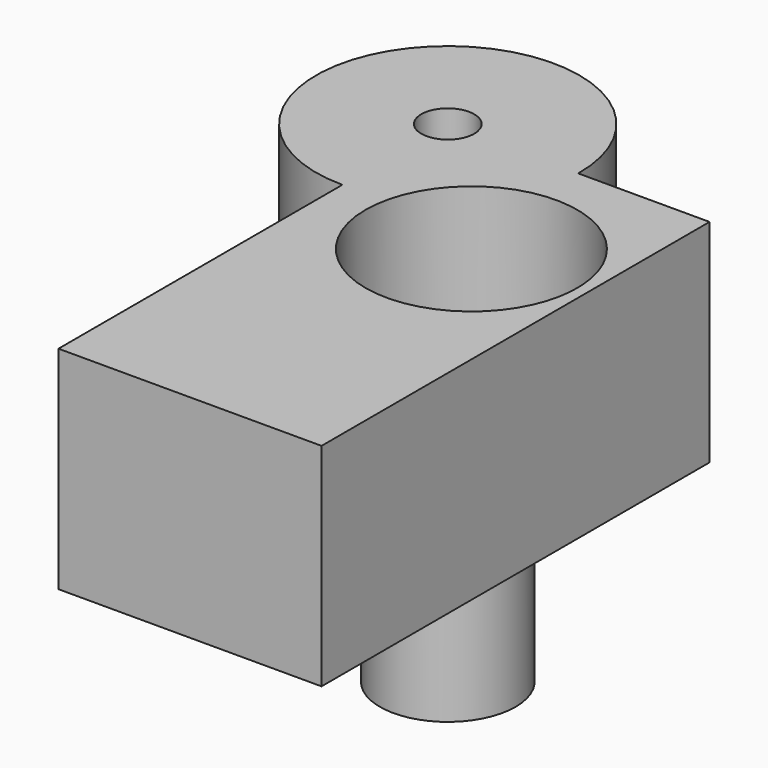
from build123d import *

# Parameters (mm, degrees)
F1_R      = 15.8036743057
F2_DEPTH  = 25.4
F0_W      = 31.5568223596
F0_H      = 33.1780388951
F3_DEPTH  = 25.4
F4_R      = 8.1334827116
F5_DEPTH  = 58.9108746499
F7_D      = 6.35
F9_D      = 25.4
F14_DEPTH = 25


# Not quite as in the source:
# - the program builds the solid bodies; features that only make, move or delete a surface that nothing else refers to are left out


with BuildPart() as f2:
    # F1 (on face) → F2 (new body)
    with BuildSketch(Plane.XY):
        with Locations((0, 33.3719775081)):
            Circle(F1_R)
    extrude(amount=F2_DEPTH)

    # F0 (on Top) → F3 (join)
    with BuildSketch(Plane.XY):
        with Locations((15.7784111798, 16.5890194476)):
            Rectangle(F0_W, F0_H)
    extrude(amount=F3_DEPTH)

    # F4 (on face) → F5 (join)
    with BuildSketch(Plane.XY.offset(25.4)):
        with Locations((0, 33.3719775081)):
            Circle(F4_R)
    extrude(amount=-F5_DEPTH)

    # F7 (through all)
    with Locations(Plane.XY.offset(25.4)):
        with Locations((0, 33.3719775081)):
            Hole(F7_D / 2)

    # F9 (through all)
    with Locations(Plane.XY.offset(25.4)):
        with Locations((17.5604298711, 14.967338182)):
            Hole(F9_D / 2)

    # F14 (add): a face of the model
    f14_faces = [f2.faces().sort_by_distance(p)[0] for p in [
        (15.7784111798, 0, 12.7),
    ]]
    extrude(f14_faces, amount=F14_DEPTH)


solid = f2.part
